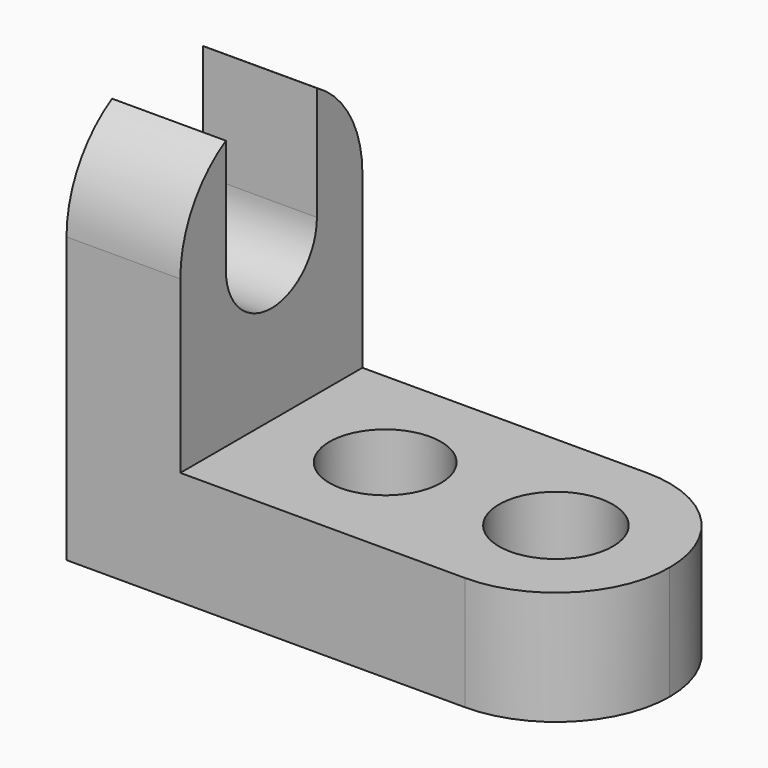
from build123d import *

# Parameters (mm, degrees)
F1_DEPTH  = 25.4
F2_R      = 6.2243902107
F2_R_2    = 6.3495156859
F3_DEPTH  = 12.701
F6_DEPTH  = 12.701
F8_DEPTH  = 12.701
F10_DEPTH = 12.701
F11_DEPTH = 12.701
F12_DEPTH = 12.701


# Not quite as in the source:
# - a feature names something its author has since deleted; it is built from what else it names


with BuildPart() as f1:
    # F0 (on Front) → F1 (new body)
    with BuildSketch(Plane.XZ):
        Polygon((-18.3063060958, 44.45), (-31.0063060958, 44.45), (-31.0063060958, 0), (26.1436939042, 0), (26.1436939042, 12.7), (-18.3063060958, 12.7), align=None)
    extrude(amount=F1_DEPTH)

    # F2 (on face) → F3 (cut, through all)
    with BuildSketch(Plane.XY.offset(12.7)):
        with Locations((-5.6063060958, -12.7)):
            Circle(F2_R)
        with Locations((13.4436939042, -12.7)):
            Circle(F2_R_2)
    extrude(amount=-F3_DEPTH, mode=Mode.SUBTRACT)

    # F4 (on face) → F6 (cut, through all)
    with BuildSketch(Plane.XY.offset(12.7)):
        with BuildLine():
            ThreePointArc((13.4436939042, 0), (22.4239500253, -3.7197438789), (26.1436939042, -12.7))
            Line((26.1436939042, -12.7), (26.1436939042, 0))
            Line((26.1436939042, 0), (13.4436939042, 0))
        make_face()
        with BuildLine():
            ThreePointArc((26.1436939042, -12.7), (22.4239500253, -21.6802561211), (13.4436939042, -25.4))
            Line((13.4436939042, -25.4), (26.1436939042, -25.4))
            Line((26.1436939042, -25.4), (26.1436939042, -12.7))
        make_face()
    extrude(amount=-F6_DEPTH, mode=Mode.SUBTRACT)

    # F7 (on face) → F8 (cut, through all)
    with BuildSketch(Plane.YZ.offset(-18.3063060958)):
        with BuildLine():
            ThreePointArc((-12.7, 44.45), (-3.7197438789, 40.7302561211), (0, 31.75))
            Line((0, 31.75), (0, 44.45))
            Line((0, 44.45), (-12.7, 44.45))
        make_face()
        with BuildLine():
            ThreePointArc((-25.4, 31.75), (-21.6802561211, 40.7302561211), (-12.7, 44.45))
            Line((-12.7, 44.45), (-25.4, 44.45))
            Line((-25.4, 44.45), (-25.4, 31.75))
        make_face()
    extrude(amount=-F8_DEPTH, mode=Mode.SUBTRACT)

    # F9 (on face) → F10 (cut, through all)
    with BuildSketch(Plane.YZ.offset(-18.3063060958)):
        with BuildLine():
            ThreePointArc((-12.7, 44.45), (-15.9870018728, 44.0172579939), (-19.05, 42.7485226281))
            Line((-19.05, 42.7485226281), (-19.05, 30.0485226281))
            ThreePointArc((-19.05, 30.0485226281), (-12.7, 23.6985226281), (-6.35, 30.0485226281))
            Line((-6.35, 30.0485226281), (-6.35, 42.7485226281))
            ThreePointArc((-6.35, 42.7485226281), (-9.4129981272, 44.0172579939), (-12.7, 44.45))
        make_face()
    extrude(amount=-F10_DEPTH, mode=Mode.SUBTRACT)

    # F7 (on face) → F11 (cut, through all)
    with BuildSketch(Plane.YZ.offset(-18.3063060958)):
        with BuildLine():
            ThreePointArc((-12.7, 44.45), (-3.7197438789, 40.7302561211), (0, 31.75))
            Line((0, 31.75), (0, 44.45))
            Line((0, 44.45), (-12.7, 44.45))
        make_face()
    extrude(amount=-F11_DEPTH, mode=Mode.SUBTRACT)

    # F7 (on face) → F12 (cut, through all)
    with BuildSketch(Plane.YZ.offset(-18.3063060958)):
        with BuildLine():
            ThreePointArc((-25.4, 31.75), (-21.6802561211, 40.7302561211), (-12.7, 44.45))
            Line((-12.7, 44.45), (-25.4, 44.45))
            Line((-25.4, 44.45), (-25.4, 31.75))
        make_face()
        with BuildLine():
            ThreePointArc((-12.7, 44.45), (-3.7197438789, 40.7302561211), (0, 31.75))
            Line((0, 31.75), (0, 44.45))
            Line((0, 44.45), (-12.7, 44.45))
        make_face()
    extrude(amount=-F12_DEPTH, mode=Mode.SUBTRACT)


solid = f1.part
